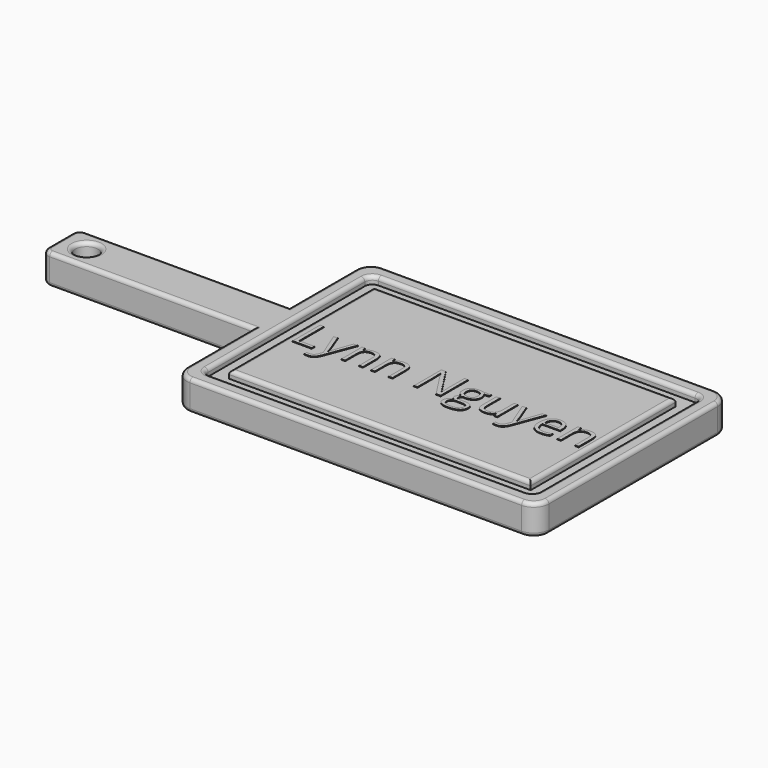
from build123d import *

# Parameters (mm, degrees)
F0_W          = 177.8
F0_H          = 38.1
F1_DEPTH      = 25.4
F2_R          = 9.525
F3_DEPTH      = 25.4
F4_W          = 279.4
F4_H          = 177.8
F4_W_2        = 254
F4_H_2        = 152.4
F5_DEPTH      = 6.35
F6_R          = 6.35
F7_R          = 12.7
F8_R          = 3.175
F10_T1_DEPTH  = 25.4
F10_T4_ANGLE  = 90
F10_T6_ANGLE  = 90
F10_T8_ANGLE  = 90
F10_T10_ANGLE = 90
F9_TEXT_SIZE  = 40.6723292874
F11_DEPTH     = 0.508


# Not quite as in the source:
# - a fillet or chamfer that OpenCascade refuses, or shapes differently, is made with other operations: its cross-section is extruded or revolved along the edge and cut away or added
# - Text() gives the source's letters only with a copy of the font that has no kerning and outlines rounded to 1/6400 em; it was checked with that copy


with BuildPart() as f1:
    # F0 (on Top) → F1 (new body)
    with BuildSketch(Plane.XY):
        Polygon((0, 82.55), (0, 0), (304.8, 0), (304.8, 203.2), (0, 203.2), (0, 120.65), align=None)
        with Locations((-88.9, 101.6)):
            Rectangle(F0_W, F0_H)
    extrude(amount=F1_DEPTH)

    # F2 (on face) → F3 (cut)
    with BuildSketch(Plane.XY.offset(25.4)):
        with Locations((-155.575, 101.6)):
            Circle(F2_R)
    extrude(amount=-F3_DEPTH, mode=Mode.SUBTRACT)

    # F4 (on face) → F5 (cut)
    with BuildSketch(Plane.XY.offset(25.4)):
        with Locations((152.4, 101.6)):
            Rectangle(F4_W, F4_H)
        with Locations((152.4, 101.6)):
            Rectangle(F4_W_2, F4_H_2, mode=Mode.SUBTRACT)
    extrude(amount=-F5_DEPTH, mode=Mode.SUBTRACT)

    # F6
    f6_edges = [f1.edges().sort_by_distance(p)[0] for p in [
        (12.7, 190.5, 22.225),
        (12.7, 12.7, 22.225),
        (292.1, 190.5, 22.225),
        (292.1, 12.7, 22.225),
    ]]
    fillet(f6_edges, radius=F6_R)

    # F7
    f7_edges = [f1.edges().sort_by_distance(p)[0] for p in [
        (304.8, 203.2, 12.7),
        (0, 203.2, 12.7),
        (0, 0, 12.7),
        (304.8, 0, 12.7),
    ]]
    fillet(f7_edges, radius=F7_R)

    # F8
    f8_edges = [f1.edges().sort_by_distance(p)[0] for p in [
        (25.4, 101.6, 25.4),
        (152.4, 177.8, 25.4),
        (279.4, 101.6, 25.4),
        (152.4, 25.4, 25.4),
        (0, 47.625, 25.4),
        (3.719744, 3.719744, 25.4),
        (-88.9, 82.55, 25.4),
        (152.4, 0, 25.4),
        (-177.8, 101.6, 25.4),
        (301.080256, 3.719744, 25.4),
        (-88.9, 120.65, 25.4),
        (304.8, 101.6, 25.4),
        (0, 155.575, 25.4),
        (301.080256, 199.480256, 25.4),
        (3.719744, 199.480256, 25.4),
        (152.4, 203.2, 25.4),
        (152.4, 190.5, 25.4),
        (290.240128, 188.640128, 25.4),
        (14.559872, 188.640128, 25.4),
        (292.1, 101.6, 25.4),
        (12.7, 101.6, 25.4),
        (290.240128, 14.559872, 25.4),
        (14.559872, 14.559872, 25.4),
        (152.4, 12.7, 25.4),
        (-165.1, 101.6, 25.4),
        (0, 47.625, 0),
        (3.719744, 3.719744, 0),
        (-88.9, 82.55, 0),
        (152.4, 0, 0),
        (-177.8, 101.6, 0),
        (301.080256, 3.719744, 0),
        (-88.9, 120.65, 0),
        (304.8, 101.6, 0),
        (0, 155.575, 0),
        (301.080256, 199.480256, 0),
        (3.719744, 199.480256, 0),
        (152.4, 203.2, 0),
        (-165.1, 101.6, 0),
    ]]
    fillet(f8_edges, radius=F8_R)

    # F10: fillet of radius 6.35 on 2 edges, made by hand

    # F10_s2 → F10_t1 (cut)
    with BuildSketch(Plane.XY):
        with BuildLine():
            ThreePointArc((-171.45, 82.55), (-175.9401280605, 84.4098719395), (-177.8, 88.9))
            Line((-177.8, 88.9), (-177.8, 82.55))
            Line((-177.8, 82.55), (-171.45, 82.55))
        make_face()
        with BuildLine():
            ThreePointArc((-177.8, 114.3), (-175.9401280605, 118.7901280605), (-171.45, 120.65))
            Line((-171.45, 120.65), (-177.8, 120.65))
            Line((-177.8, 120.65), (-177.8, 114.3))
        make_face()
    extrude(amount=F10_T1_DEPTH, mode=Mode.SUBTRACT)

    # F10_s3 → F10_t4 (revolve, cut)
    with BuildSketch(Plane.XZ.offset(-114.3)):
        with BuildLine():
            ThreePointArc((-174.625, 0), (-176.8700640303, 0.9299359697), (-177.8, 3.175))
            Line((-177.8, 3.175), (-177.8, 0))
            Line((-177.8, 0), (-174.625, 0))
        make_face()
    revolve(axis=Axis((-171.45, 114.3, 0), (0, 0, -1)), revolution_arc=F10_T4_ANGLE, mode=Mode.SUBTRACT)

    # F10_s5 → F10_t6 (revolve, cut)
    with BuildSketch(Plane.YZ.offset(-171.45)):
        with BuildLine():
            ThreePointArc((117.475, 25.4), (119.7200640303, 24.4700640303), (120.65, 22.225))
            Line((120.65, 22.225), (120.65, 25.4))
            Line((120.65, 25.4), (117.475, 25.4))
        make_face()
    revolve(axis=Axis((-171.45, 114.3, 25.4), (0, 0, 1)), revolution_arc=F10_T6_ANGLE, mode=Mode.SUBTRACT)

    # F10_s7 → F10_t8 (revolve, cut)
    with BuildSketch(Plane.YZ.offset(-171.45)):
        with BuildLine():
            ThreePointArc((85.725, 0), (83.4799359697, 0.9299359697), (82.55, 3.175))
            Line((82.55, 3.175), (82.55, 0))
            Line((82.55, 0), (85.725, 0))
        make_face()
    revolve(axis=Axis((-171.45, 88.9, 0), (0, 0, -1)), revolution_arc=F10_T8_ANGLE, mode=Mode.SUBTRACT)

    # F10_s9 → F10_t10 (revolve, cut)
    with BuildSketch(Plane.XZ.offset(-88.9)):
        with BuildLine():
            ThreePointArc((-174.625, 25.4), (-176.8700640303, 24.4700640303), (-177.8, 22.225))
            Line((-177.8, 22.225), (-177.8, 25.4))
            Line((-177.8, 25.4), (-174.625, 25.4))
        make_face()
    revolve(axis=Axis((-171.45, 88.9, 25.4), (0, 0, 1)), revolution_arc=F10_T10_ANGLE, mode=Mode.SUBTRACT)

    # F9 (on face) → F11 (join)
    with BuildSketch(Plane.XY.offset(25.4)):
        with Locations((28.575, 83.1485582064)):
            Text('Lynn Nguyen', F9_TEXT_SIZE, font='Open Sans', text_align=(TextAlign.LEFT, TextAlign.BOTTOM))
    extrude(amount=F11_DEPTH)


solid = f1.part
